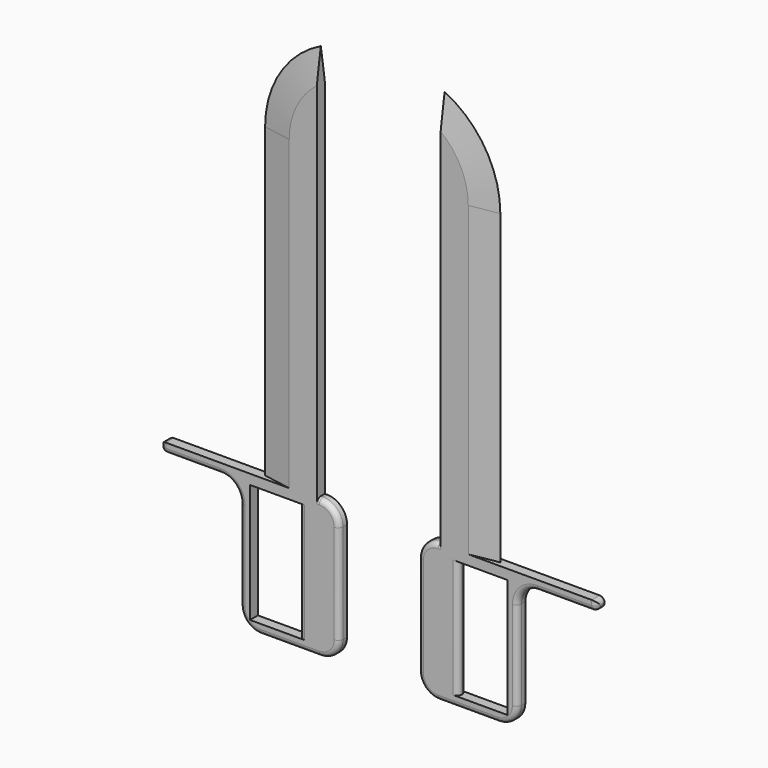
from build123d import *

# Parameters (mm, degrees)
F0_W        = 101.6
F0_H        = 12.7
F1_DEPTH    = 12.7
F3_DEPTH    = 12.7
F4_T1_DEPTH = 583.7036907444
F5_R        = 6.34999
F6_R        = 25.4
F7_R        = 6.35
F8_R        = 6.34999
F9_SIZE2    = 36.01263
F9_SIZE     = 6.34999


# Not quite as in the source:
# - a fillet or chamfer that OpenCascade refuses, or shapes differently, is made with other operations: its cross-section is extruded or revolved along the edge and cut away or added
# - a fillet or chamfer is up to 0.001 mm smaller than in the source, because OpenCascade refuses the exact size


with BuildPart() as f1:
    # F0 (on Front) → F1 (new body)
    with BuildSketch(Plane.XZ):
        Polygon((-50.8, -88.9), (-50.8, -76.2), (-101.6, -76.2), (-165.1, -76.2), (-165.1, 76.2), (-177.8, 76.2), (-177.8, -88.9), align=None)
        Polygon((-101.6, -76.2), (-50.8, -76.2), (-50.8, 0), (-50.8, 76.2), (-101.6, 76.2), align=None)
        Polygon((-165.1, 76.2), (-101.6, 76.2), (-50.8, 76.2), (-50.8, 88.9), (-177.8, 88.9), (-177.8, 76.2), align=None)
        with Locations((-228.6, 82.55)):
            Rectangle(F0_W, F0_H)
    extrude(amount=F1_DEPTH)

    # F2 (on face) → F3 (join)
    with BuildSketch(Plane.XZ.offset(12.7)):
        Polygon((-107.95, 88.9), (-79.375, 88.9), (-79.375, 596.9), (-150.8125, 596.9), (-150.8125, 88.9), (-136.525, 88.9), align=None)
    extrude(amount=-F3_DEPTH)

    # F4: fillet of radius 127 on 1 edges, made by hand

    # F4_s2 → F4_t1 (cut)
    with BuildSketch(Plane.XZ.offset(-285.5018453722)):
        with BuildLine():
            ThreePointArc((-79.375, 596.9), (-131.4819884821, 550.0511827591), (-150.8125, 482.6992618511))
            Line((-150.8125, 482.6992618511), (-150.8125, 596.9))
            Line((-150.8125, 596.9), (-79.375, 596.9))
        make_face()
    extrude(amount=F4_T1_DEPTH, mode=Mode.SUBTRACT)

    # F5 (radius 6.35 in the source; OpenCascade refuses exactly that, so slightly less here)
    f5_edges = [f1.edges().sort_by_distance(p)[0] for p in [
        (-101.6, -12.7, 0),
        (-101.6, 0, 0),
    ]]
    fillet(f5_edges, radius=F5_R)

    # F6
    f6_edges = [f1.edges().sort_by_distance(p)[0] for p in [
        (-50.8, -6.35, 88.9),
        (-50.8, -6.35, -88.9),
        (-177.8, -6.35, -88.9),
        (-177.8, -6.35, 76.2),
    ]]
    fillet(f6_edges, radius=F6_R)

    # F7
    f7_edges = [f1.edges().sort_by_distance(p)[0] for p in [
        (-50.8, -12.7, 0),
    ]]
    fillet(f7_edges, radius=F7_R)

    # F8 (radius 6.35 in the source; OpenCascade refuses exactly that, so slightly less here)
    f8_edges = [f1.edges().sort_by_distance(p)[0] for p in [
        (-279.4, -12.7, 85.725),
        (-279.4, -6.35, 88.9),
        (-279.4, -3.175, 76.2),
        (-279.4, -10.840128, 78.059872),
    ]]
    fillet(f8_edges, radius=F8_R)

    # F9 (size 6.35 and 36.0126395546 in the source; OpenCascade refuses exactly that, so slightly less here)
    f9_edges = [f1.edges().sort_by_distance(p)[0] for p in [
        (-150.8125, -12.7, 285.799631),
        (-150.8125, 0, 285.799631),
    ]]
    f9_side = f1.faces().sort_by_distance((-150.8125, -6.35, 285.799631))[0]
    chamfer(f9_edges, length=F9_SIZE, length2=F9_SIZE2, reference=f9_side)


with BuildPart() as f10_1:
    # F10: instance of F1
    add(f1.part.mirror(Plane.YZ))


solid = Compound([f1.part, f10_1.part])
